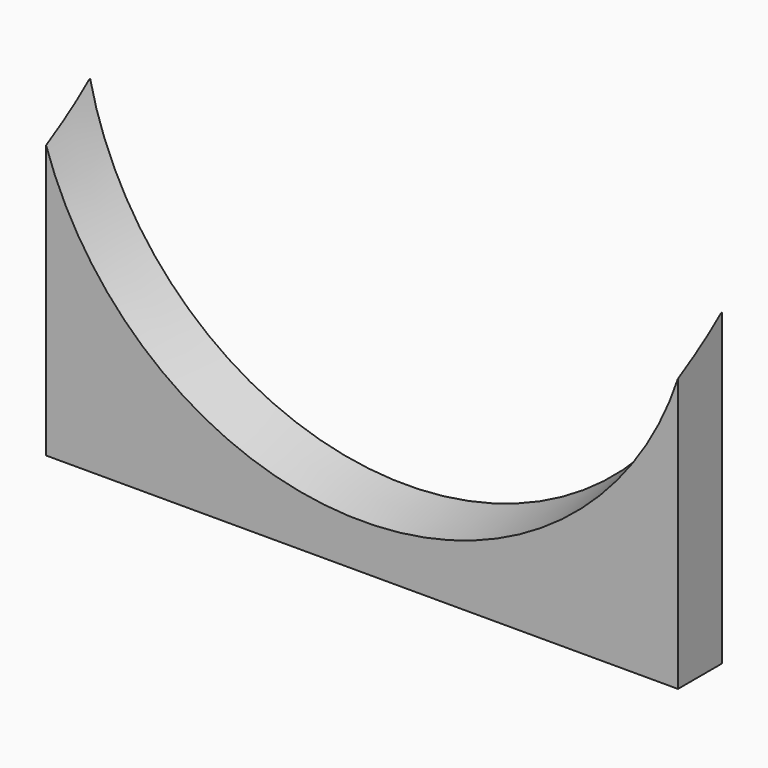
from build123d import *

# Parameters (mm, degrees)
F1_DEPTH    = 10.16
F2_T2_ANGLE = 284.1697303729


# Not quite as in the source:
# - a fillet or chamfer that OpenCascade refuses, or shapes differently, is made with other operations: its cross-section is extruded or revolved along the edge and cut away or added


with BuildPart() as f1:
    # F0 (on Front) → F1 (new body)
    with BuildSketch(Plane.XZ):
        with BuildLine():
            Line((-116.84, 0), (0, 0))
            Line((0, 0), (0, 57.15))
            Line((0, 57.15), (-2.6989761401, 57.15))
            ThreePointArc((-2.6989761401, 57.15), (-58.42, 12.7), (-114.1410238599, 57.15))
            Line((-114.1410238599, 57.15), (-116.84, 57.15))
            Line((-116.84, 57.15), (-116.84, 0))
        make_face()
    extrude(amount=F1_DEPTH)

    # F2: chamfer of 24.892 x 4.3891312038 on 1 edges, made by hand

    # F2_s1 → F2_t2 (revolve, cut)
    with BuildSketch(Plane(origin=(-70.2228677722, 0, 54.6968082658), x_dir=(0, 1, 0), z_dir=(-0.7889217924, 0, 0.6144936171))):
        Polygon((14.732, -76.3574700932), (-10.16, -80.746601297), (-10.16, -76.3574700932), align=None)
    revolve(axis=Axis((-58.42, -10.16, 69.85), (0, 1, 0)), revolution_arc=F2_T2_ANGLE, mode=Mode.SUBTRACT)


solid = f1.part
